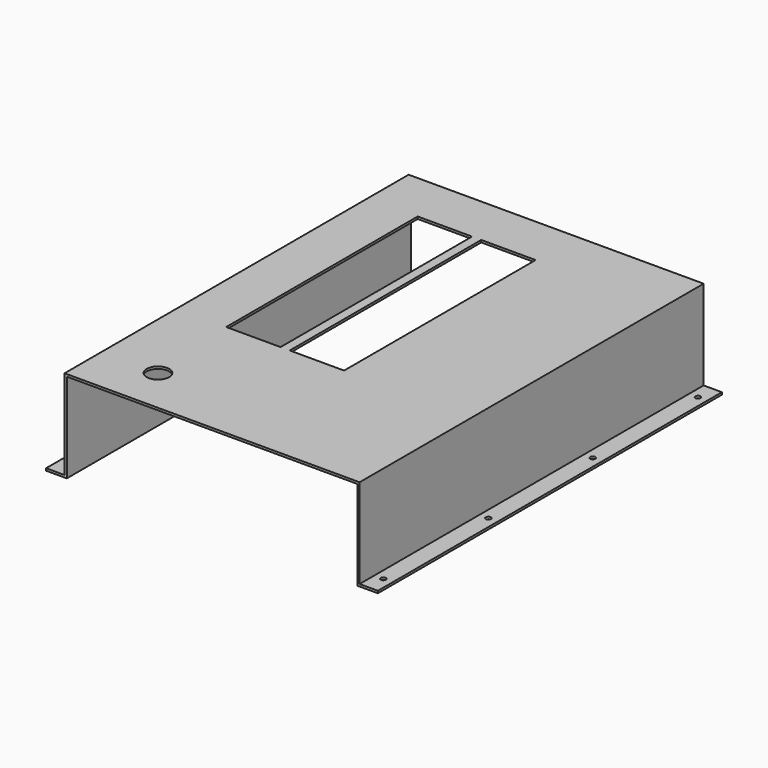
from build123d import *

# Parameters (mm, degrees)
F1_DEPTH = 609.092
F2_W     = 77
F2_H     = 339
F3_DEPTH = 25.4
F4_R     = 15.875
F5_DEPTH = 25.4
F7_D     = 7.14375


# Not quite as in the source:
# - a length typed as a fraction of an inch, garbled in the dataset ("3 / 203.2 mm" for 3/8 in), is restored


with BuildPart() as f1:
    # F0 (on Front) → F1 (new body)
    with BuildSketch(Plane.XZ):
        Polygon((0, -3.175), (0, 0), (-25.908, 0), (-25.908, 126.873), (-443.738, 126.873), (-443.738, 0), (-469.9, 0), (-469.9, -3.175), (-440.563, -3.175), (-440.563, 123.698), (-29.083, 123.698), (-29.083, -3.175), align=None)
    extrude(amount=F1_DEPTH)

    # F2 (on face) → F3 (cut)
    with BuildSketch(Plane.XY.offset(126.873)):
        with Locations((-334.88, -241.382)):
            Rectangle(F2_W, F2_H)
        with Locations((-244.88, -241.382)):
            Rectangle(F2_W, F2_H)
    extrude(amount=-F3_DEPTH, mode=Mode.SUBTRACT)

    # F4 (on face) → F5 (cut)
    with BuildSketch(Plane.XY.offset(126.873)):
        with Locations((-363.474, -544.068)):
            Circle(F4_R)
    extrude(amount=-F5_DEPTH, mode=Mode.SUBTRACT)

    # F7 (through all)
    with Locations(Plane.XY):
        with Locations((-456.946, -25.908), (-456.946, -212.09), (-456.946, -397.002), (-456.946, -582.93), (-13.208, -582.93), (-13.208, -397.002), (-13.208, -212.09), (-13.208, -25.908)):
            Hole(F7_D / 2)


solid = f1.part
